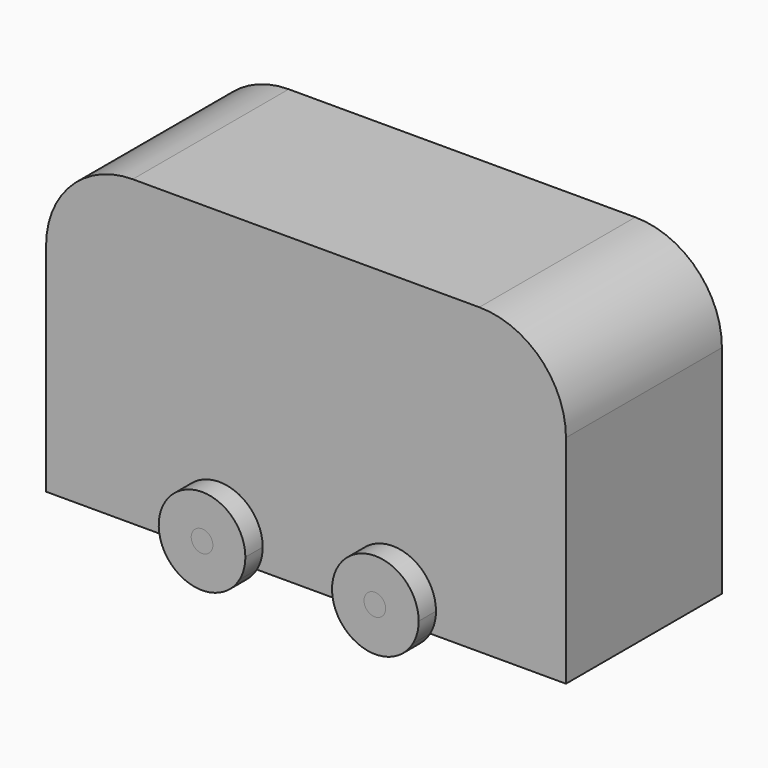
from build123d import *

# Parameters (mm, degrees)
F1_DEPTH    = 28.575
F3_DEPTH    = 6.35
F4_R        = 3.175
F5_DEPTH    = 6.35
F6_R        = 3.175
F5_FACE_R   = 12.7
F5_FACE_R_2 = 3.175
F7_DEPTH    = 69.851
F8_DEPTH    = 69.85


# Not quite as in the source:
# - a feature names something its author has since deleted; it is built from what else it names


with BuildPart() as f1:
    # F0 (on Front) → F1 (new body, symmetric)
    with BuildSketch(Plane.XZ):
        with BuildLine():
            Line((-76.2, -44.45), (76.2, -44.45))
            Line((76.2, -44.45), (76.2, 19.05))
            ThreePointArc((76.2, 19.05), (68.7605122421, 37.0105122421), (50.8, 44.45))
            Line((50.8, 44.45), (-50.8, 44.45))
            ThreePointArc((-50.8, 44.45), (-68.7605122421, 37.0105122421), (-76.2, 19.05))
            Line((-76.2, 19.05), (-76.2, -44.45))
        make_face()
    extrude(amount=F1_DEPTH, both=True)

    # F4 (on face) → F5 (join)
    with BuildSketch(Plane(origin=(0, 28.575, 0), x_dir=(-1, 0, 0), z_dir=(0, 1, 0))):
        with BuildLine():
            Line((-14.4014773719, -44.45), (-36.3985226281, -44.45))
            ThreePointArc((-36.3985226281, -44.45), (-25.4, -50.8), (-14.4014773719, -44.45))
        make_face()
        with BuildLine():
            ThreePointArc((38.1, -38.1), (22.1129981272, -25.8327420061), (14.4014773719, -44.45))
            Line((14.4014773719, -44.45), (36.3985226281, -44.45))
            ThreePointArc((36.3985226281, -44.45), (37.6672579939, -41.3870018728), (38.1, -38.1))
        make_face()
        with Locations((25.4, -38.1)):
            Circle(F4_R, mode=Mode.SUBTRACT)
        with BuildLine():
            Line((36.3985226281, -44.45), (14.4014773719, -44.45))
            ThreePointArc((14.4014773719, -44.45), (25.4, -50.8), (36.3985226281, -44.45))
        make_face()
        with BuildLine():
            ThreePointArc((-14.4014773719, -44.45), (-13.1327420061, -41.3870018728), (-12.7, -38.1))
            ThreePointArc((-12.7, -38.1), (-28.6870018728, -25.8327420061), (-36.3985226281, -44.45))
            Line((-36.3985226281, -44.45), (-14.4014773719, -44.45))
        make_face()
        with Locations((-25.4, -38.1)):
            Circle(F4_R, mode=Mode.SUBTRACT)
    extrude(amount=F5_DEPTH)


with BuildPart() as f3:
    # F2 (on face) → F3 (new body)
    with BuildSketch(Plane.XZ.offset(28.575)):
        with BuildLine():
            ThreePointArc((-36.3985226281, -44.45), (-25.4, -50.8), (-14.4014773719, -44.45))
            Line((-14.4014773719, -44.45), (-36.3985226281, -44.45))
        make_face()
        with BuildLine():
            Line((-36.3985226281, -44.45), (-14.4014773719, -44.45))
            ThreePointArc((-14.4014773719, -44.45), (-13.1327420061, -41.3870018728), (-12.7, -38.1))
            ThreePointArc((-12.7, -38.1), (-28.6870018728, -25.8327420061), (-36.3985226281, -44.45))
        make_face()
    extrude(amount=F3_DEPTH)


with BuildPart() as f3b:
    # F2 (on face) → F3, piece 2 (new body)
    with BuildSketch(Plane.XZ.offset(28.575)):
        with BuildLine():
            ThreePointArc((36.3985226281, -44.45), (37.6672579939, -41.3870018728), (38.1, -38.1))
            ThreePointArc((38.1, -38.1), (22.1129981272, -25.8327420061), (14.4014773719, -44.45))
            Line((14.4014773719, -44.45), (36.3985226281, -44.45))
        make_face()
        with BuildLine():
            Line((36.3985226281, -44.45), (14.4014773719, -44.45))
            ThreePointArc((14.4014773719, -44.45), (25.4, -50.8), (36.3985226281, -44.45))
        make_face()
    extrude(amount=F3_DEPTH)


with BuildPart() as f7_tool:
    # F6 (on face) + F4 (on face) + F5_face (on face) → F7 (new body, through all)
    with BuildSketch(Plane.XZ.offset(34.925)):
        with Locations((-25.4, -38.1)):
            Circle(F6_R)
        with Locations((25.2535380423, -38.0017161369)):
            Circle(F6_R)
    with BuildSketch(Plane(origin=(0, 28.575, 0), x_dir=(-1, 0, 0), z_dir=(0, 1, 0))):
        with Locations((-25.4, -38.1)):
            Circle(F4_R)
        with Locations((25.4, -38.1)):
            Circle(F4_R)
    with BuildSketch(Plane(origin=(-25.4, 34.925, -38.1), x_dir=(-1, 0, 0), z_dir=(0, 1, 0))):
        Circle(F5_FACE_R)
        Circle(F5_FACE_R_2, mode=Mode.SUBTRACT)
        with Locations((-50.8, 0)):
            Circle(F5_FACE_R)
        with Locations((-50.8, 0)):
            Circle(F5_FACE_R_2, mode=Mode.SUBTRACT)
    extrude(amount=-F7_DEPTH, dir=(0, -1, 0))


with BuildPart() as f1_1:
    add(f1.part)

    # F7: cut by f7_tool
    add(f7_tool.part, mode=Mode.SUBTRACT)


with BuildPart() as f3_1:
    add(f3.part)

    # F7: cut by f7_tool
    add(f7_tool.part, mode=Mode.SUBTRACT)


with BuildPart() as f3b_1:
    add(f3b.part)

    # F7: cut by f7_tool
    add(f7_tool.part, mode=Mode.SUBTRACT)


with BuildPart() as f8:
    # F6 (on face) → F8 (new body)
    with BuildSketch(Plane.XZ.offset(34.925)):
        with Locations((-25.4, -38.1)):
            Circle(F6_R)
    extrude(amount=-F8_DEPTH)


with BuildPart() as f8b:
    # F6 (on face) → F8, piece 2 (new body)
    with BuildSketch(Plane.XZ.offset(34.925)):
        with Locations((25.2535380423, -38.0017161369)):
            Circle(F6_R)
    extrude(amount=-F8_DEPTH)


solid = Compound([f1_1.part, f3_1.part, f3b_1.part, f8.part, f8b.part])
